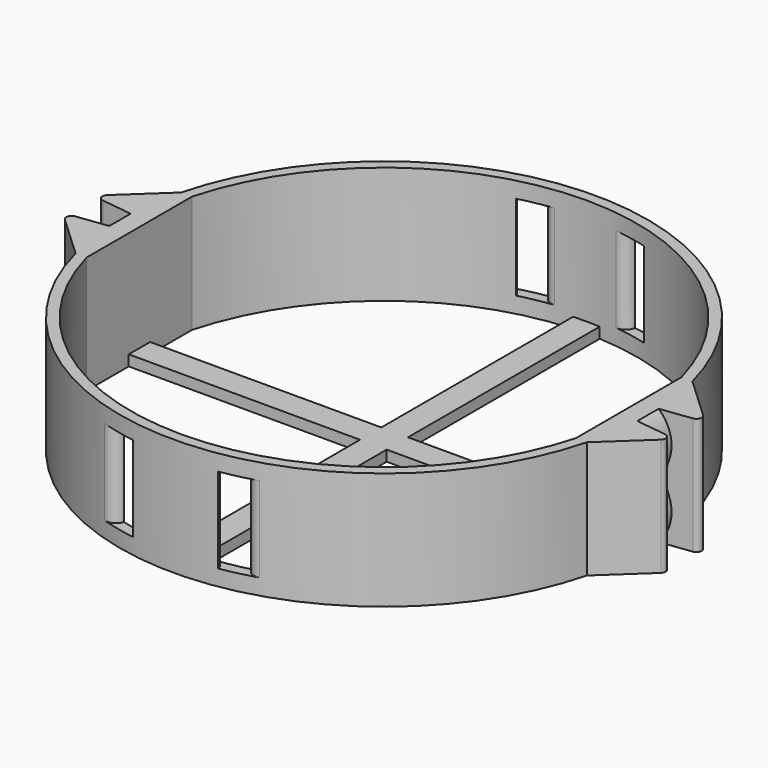
from build123d import *

# Parameters (mm, degrees)
F1_DEPTH      = 27.94
F2_W          = 59.69
F2_H          = 6.35
F2_W_2        = 6.35
F3_DEPTH      = 2.54
F4_W          = 5.08
F4_H          = 20.32
F5_DEPTH      = 62.866
F5_DEPTH_BACK = 62.866
F6_T1_DEPTH   = 20.32
F8_DEPTH      = 3.5254948624
F8_DEPTH_BACK = 3.5254948624


# Not quite as in the source:
# - a fillet or chamfer that OpenCascade refuses, or shapes differently, is made with other operations: its cross-section is extruded or revolved along the edge and cut away or added


with BuildPart() as f1:
    # F0 (on Top) → F1 (new body)
    with BuildSketch(Plane.XY):
        with BuildLine():
            Line((-70.9619581652, -6.2947835132), (-60.8714999798, -15.7056905359))
            ThreePointArc((-60.8714999798, -15.7056905359), (-62.3646336926, -7.9158505156), (-62.865, 0))
            Line((-62.865, 0), (-62.865, -3.175))
            Line((-62.865, -3.175), (-70.254501201, -4.1059896424))
            ThreePointArc((-70.254501201, -4.1059896424), (-71.304196006, -4.9754379298), (-70.9619581652, -6.2947835132))
        make_face()
        with BuildLine():
            ThreePointArc((-58.2446298794, 15.7056905359), (0, 60.325), (58.2446298794, 15.7056905359))
            Line((58.2446298794, 15.7056905359), (60.8714999798, 15.7056905359))
            ThreePointArc((60.8714999798, 15.7056905359), (0, 62.865), (-60.8714999798, 15.7056905359))
            Line((-60.8714999798, 15.7056905359), (-58.2446298794, 15.7056905359))
        make_face()
        with BuildLine():
            ThreePointArc((-58.2446298794, -15.7056905359), (-60.325, 0), (-58.2446298794, 15.7056905359))
            Line((-58.2446298794, 15.7056905359), (-60.8714999798, 15.7056905359))
            ThreePointArc((-60.8714999798, 15.7056905359), (-62.3646336926, 7.9158505156), (-62.865, 0))
            ThreePointArc((-62.865, 0), (-62.3646336926, -7.9158505156), (-60.8714999798, -15.7056905359))
            Line((-60.8714999798, -15.7056905359), (-58.2446298794, -15.7056905359))
        make_face()
        with BuildLine():
            Line((60.8714999798, -15.7056905359), (58.2446298794, -15.7056905359))
            ThreePointArc((58.2446298794, -15.7056905359), (0, -60.325), (-58.2446298794, -15.7056905359))
            Line((-58.2446298794, -15.7056905359), (-60.8714999798, -15.7056905359))
            ThreePointArc((-60.8714999798, -15.7056905359), (0, -62.865), (60.8714999798, -15.7056905359))
        make_face()
        with BuildLine():
            ThreePointArc((58.2446298794, 15.7056905359), (59.8026459384, 7.9214369758), (60.325, 0))
            ThreePointArc((60.325, 0), (59.8026459384, -7.9214369758), (58.2446298794, -15.7056905359))
            Line((58.2446298794, -15.7056905359), (60.8714999798, -15.7056905359))
            ThreePointArc((60.8714999798, -15.7056905359), (62.3646336926, -7.9158505156), (62.865, 0))
            ThreePointArc((62.865, 0), (62.3646336926, 7.9158505156), (60.8714999798, 15.7056905359))
            Line((60.8714999798, 15.7056905359), (58.2446298794, 15.7056905359))
        make_face()
        with BuildLine():
            Line((70.9619581652, 6.2947835132), (60.8714999798, 15.7056905359))
            ThreePointArc((60.8714999798, 15.7056905359), (62.3646336926, 7.9158505156), (62.865, 0))
            Line((62.865, 0), (62.865, 3.175))
            Line((62.865, 3.175), (70.254501201, 4.1059896424))
            ThreePointArc((70.254501201, 4.1059896424), (71.304196006, 4.9754379298), (70.9619581652, 6.2947835132))
        make_face()
        with BuildLine():
            ThreePointArc((62.865, 0), (62.3646336926, -7.9158505156), (60.8714999798, -15.7056905359))
            Line((60.8714999798, -15.7056905359), (70.9619581652, -6.2947835132))
            ThreePointArc((70.9619581652, -6.2947835132), (71.304196006, -4.9754379298), (70.254501201, -4.1059896424))
            Line((70.254501201, -4.1059896424), (62.865, -3.175))
            Line((62.865, -3.175), (62.865, 0))
        make_face()
        with BuildLine():
            ThreePointArc((-62.865, 0), (-62.3646336926, 7.9158505156), (-60.8714999798, 15.7056905359))
            Line((-60.8714999798, 15.7056905359), (-70.9619581652, 6.2947835132))
            ThreePointArc((-70.9619581652, 6.2947835132), (-71.304196006, 4.9754379298), (-70.254501201, 4.1059896424))
            Line((-70.254501201, 4.1059896424), (-62.865, 3.175))
            Line((-62.865, 3.175), (-62.865, 0))
        make_face()
        with BuildLine():
            ThreePointArc((58.2446298794, -15.7056905359), (59.8026459384, -7.9214369758), (60.325, 0))
            ThreePointArc((60.325, 0), (59.8026459384, 7.9214369758), (58.2446298794, 15.7056905359))
            Line((58.2446298794, 15.7056905359), (58.2446298794, -15.7056905359))
        make_face()
        with BuildLine():
            Line((-58.2446298794, -15.7056905359), (-58.2446298794, 15.7056905359))
            ThreePointArc((-58.2446298794, 15.7056905359), (-60.325, 0), (-58.2446298794, -15.7056905359))
        make_face()
    extrude(amount=F1_DEPTH)

    # F2 (on face) → F3 (join)
    with BuildSketch(Plane(origin=(0, 0, 0), x_dir=(1, 0, 0), z_dir=(0, 0, -1))):
        with Locations((33.02, 0)):
            Rectangle(F2_W, F2_H)
        Rectangle(F2_W_2, F2_H)
        with Locations((-33.02, 0)):
            Rectangle(F2_W, F2_H)
        with BuildLine():
            Line((-3.175, 3.175), (3.175, 3.175))
            Line((3.175, 3.175), (3.175, 60.2413894262))
            ThreePointArc((3.175, 60.2413894262), (0, 60.325), (-3.175, 60.2413894262))
            Line((-3.175, 60.2413894262), (-3.175, 3.175))
        make_face()
        with BuildLine():
            Line((3.175, -60.2413894262), (3.175, -3.175))
            Line((3.175, -3.175), (-3.175, -3.175))
            Line((-3.175, -3.175), (-3.175, -60.2413894262))
            ThreePointArc((-3.175, -60.2413894262), (0, -60.325), (3.175, -60.2413894262))
        make_face()
    extrude(amount=-F3_DEPTH)

    # F4 (on Front) → F5 (cut, two sides)
    with BuildSketch(Plane.XZ) as f5_sk:
        with Locations((-12.7, 13.97)):
            Rectangle(F4_W, F4_H)
        with Locations((12.7, 13.97)):
            Rectangle(F4_W, F4_H)
    extrude(amount=-F5_DEPTH, mode=Mode.SUBTRACT)
    extrude(f5_sk.sketch, amount=F5_DEPTH_BACK, mode=Mode.SUBTRACT)

    # F6: fillet of radius 2.54 on 8 edges, made by hand

    # F6_s2 → F6_t1 (cut)
    with BuildSketch(Plane.XY.offset(3.81)):
        with BuildLine():
            ThreePointArc((18.4281257881, 60.1033477016), (16.4693425511, 59.9059132544), (15.24, 58.3682107401))
            Line((15.24, 58.3682107401), (15.24, 60.9897583615))
            ThreePointArc((15.24, 60.9897583615), (16.8398962136, 60.5675335515), (18.4281257881, 60.1033477016))
        make_face()
        with BuildLine():
            ThreePointArc((-18.4281257881, 60.1033477016), (-16.4693425511, 59.9059132544), (-15.24, 58.3682107401))
            Line((-15.24, 58.3682107401), (-15.24, 60.9897583615))
            ThreePointArc((-15.24, 60.9897583615), (-16.8398962136, 60.5675335515), (-18.4281257881, 60.1033477016))
        make_face()
        with BuildLine():
            ThreePointArc((7.3366965941, 59.8771952256), (9.1895995283, 60.3814871069), (10.16, 62.038557567))
            Line((10.16, 62.038557567), (10.16, 59.4632661817))
            ThreePointArc((10.16, 59.4632661817), (8.7507960918, 59.6869264811), (7.3366965941, 59.8771952256))
        make_face()
        with BuildLine():
            ThreePointArc((-7.3366965941, 59.8771952256), (-9.1895995283, 60.3814871069), (-10.16, 62.038557567))
            Line((-10.16, 62.038557567), (-10.16, 59.4632661817))
            ThreePointArc((-10.16, 59.4632661817), (-8.7507960918, 59.6869264811), (-7.3366965941, 59.8771952256))
        make_face()
        with BuildLine():
            ThreePointArc((-18.4281257881, -60.1033477016), (-16.4693425511, -59.9059132544), (-15.24, -58.3682107401))
            Line((-15.24, -58.3682107401), (-15.24, -60.9897583615))
            ThreePointArc((-15.24, -60.9897583615), (-16.8398962136, -60.5675335515), (-18.4281257881, -60.1033477016))
        make_face()
        with BuildLine():
            ThreePointArc((18.4281257881, -60.1033477016), (16.4693425511, -59.9059132544), (15.24, -58.3682107401))
            Line((15.24, -58.3682107401), (15.24, -60.9897583615))
            ThreePointArc((15.24, -60.9897583615), (16.8398962136, -60.5675335515), (18.4281257881, -60.1033477016))
        make_face()
        with BuildLine():
            ThreePointArc((7.3366965941, -59.8771952256), (9.1895995283, -60.3814871069), (10.16, -62.038557567))
            Line((10.16, -62.038557567), (10.16, -59.4632661817))
            ThreePointArc((10.16, -59.4632661817), (8.7507960918, -59.6869264811), (7.3366965941, -59.8771952256))
        make_face()
        with BuildLine():
            ThreePointArc((-7.3366965941, -59.8771952256), (-9.1895995283, -60.3814871069), (-10.16, -62.038557567))
            Line((-10.16, -62.038557567), (-10.16, -59.4632661817))
            ThreePointArc((-10.16, -59.4632661817), (-8.7507960918, -59.6869264811), (-7.3366965941, -59.8771952256))
        make_face()
    extrude(amount=F6_T1_DEPTH, mode=Mode.SUBTRACT)

    # F7 (on Front) → F8 (join, two sides)
    with BuildSketch(Plane.XZ) as f8_sk:
        with BuildLine():
            ThreePointArc((65.0278285183, 17.4625), (65.4371804989, 23.0089829265), (62.865, 27.94))
            Line((62.865, 27.94), (62.865, 0))
            ThreePointArc((62.865, 0), (65.4371804989, 4.9310170735), (65.0278285183, 10.4775))
            ThreePointArc((65.0278285183, 10.4775), (64.4086903111, 13.97), (65.0278285183, 17.4625))
        make_face()
        with BuildLine():
            ThreePointArc((-65.0278285183, 10.4775), (-65.4371804989, 4.9310170735), (-62.865, 0))
            Line((-62.865, 0), (-62.865, 27.94))
            ThreePointArc((-62.865, 27.94), (-65.4371804989, 23.0089829265), (-65.0278285183, 17.4625))
            ThreePointArc((-65.0278285183, 17.4625), (-64.4086903111, 13.97), (-65.0278285183, 10.4775))
        make_face()
    extrude(amount=F8_DEPTH)
    extrude(f8_sk.sketch, amount=-F8_DEPTH_BACK)


solid = f1.part
